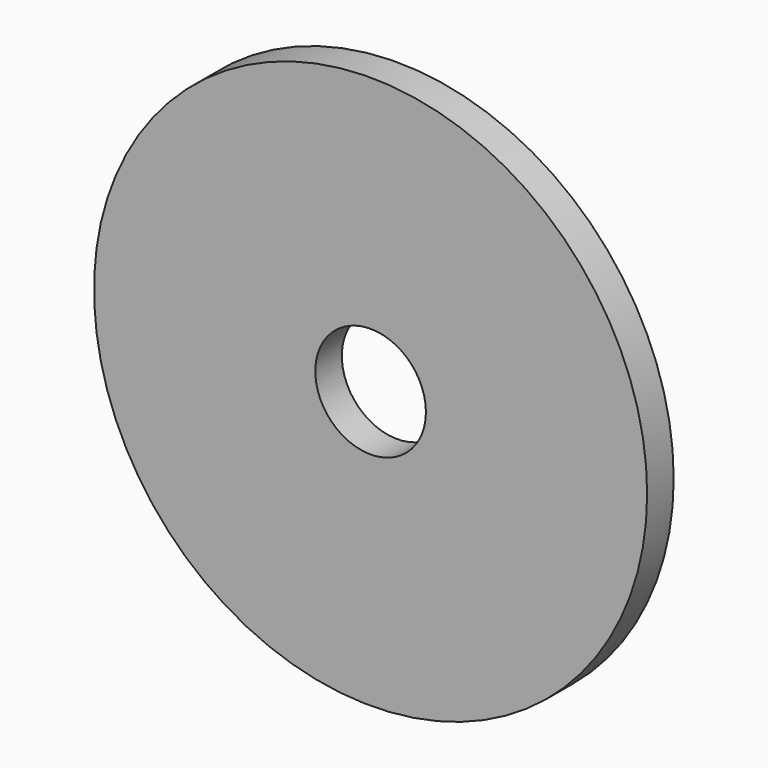
from build123d import *

# Parameters (mm, degrees)
F0_R     = 63.5
F0_R_2   = 12.7
F1_DEPTH = 3.81


# Not quite as in the source:
# - the program builds the solid bodies; features that only make, move or delete a surface that nothing else refers to are left out


with BuildPart() as f1:
    # F0 (on Front) → F1 (new body, symmetric)
    with BuildSketch(Plane.XZ):
        Circle(F0_R)
        Circle(F0_R_2, mode=Mode.SUBTRACT)
    extrude(amount=F1_DEPTH, both=True)


solid = f1.part
